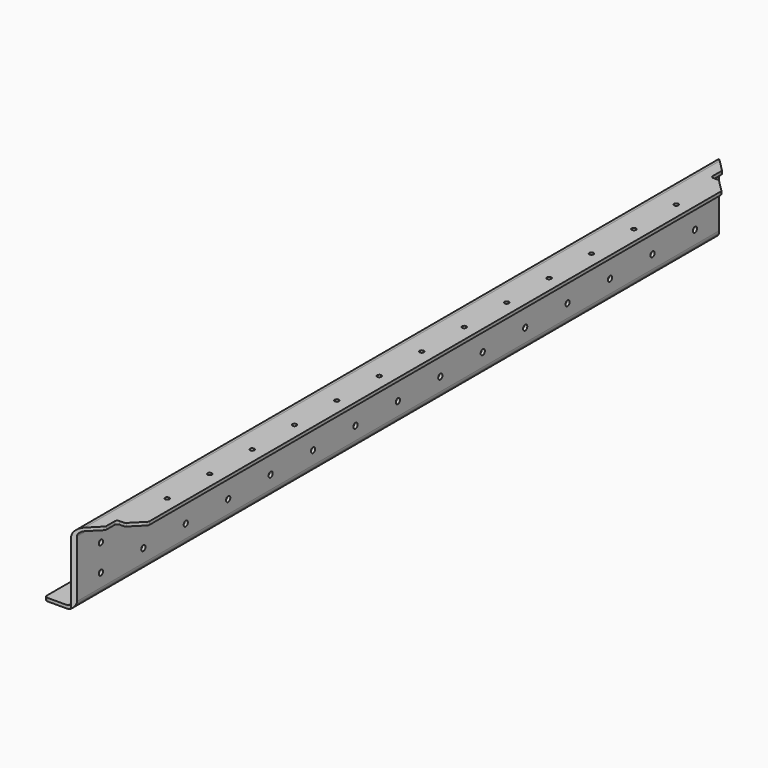
from build123d import *

# Parameters (mm, degrees)
F1_DEPTH    = 1525
F3_DEPTH    = 136.001
F4_R        = 8
F5_R        = 8
F6_R        = 14
F7_T1_DEPTH = 1583
F8_R        = 4.1
F9_DEPTH    = 136.001
F10_R       = 5
F11_DEPTH   = 76.001
F12_R       = 5
F13_DEPTH   = 6.001
F15_DEPTH   = 136.001
F16_R       = 5


# Not quite as in the source:
# - a fillet or chamfer that OpenCascade refuses, or shapes differently, is made with other operations: its cross-section is extruded or revolved along the edge and cut away or added
# - two fillets or chamfers of one size are made in one step


with BuildPart() as f1:
    # F0 (on Front) → F1 (new body)
    with BuildSketch(Plane.XZ):
        Polygon((0, 130), (0, 0), (-50, 0), (-50, -6), (6, -6), (6, 124), (76, 124), (76, 130), align=None)
    extrude(amount=F1_DEPTH)

    # F2 (on face) → F3 (cut, through all)
    with BuildSketch(Plane.XY.offset(130)):
        Polygon((76, -76), (76, 0), (0, 0), align=None)
        Polygon((76, -1525), (76, -1449), (0, -1525), align=None)
    extrude(amount=-F3_DEPTH, mode=Mode.SUBTRACT)

    # F4
    f4_edges = [f1.edges().sort_by_distance(p)[0] for p in [
        (6, -762.5, 124),
    ]]
    fillet(f4_edges, radius=F4_R)

    # F5
    f5_edges = [f1.edges().sort_by_distance(p)[0] for p in [
        (0, -762.5, 0),
    ]]
    fillet(f5_edges, radius=F5_R)

    # F6
    f6_edges = [f1.edges().sort_by_distance(p)[0] for p in [
        (0, -762.5, 130),
    ]]
    fillet(f6_edges, radius=F6_R)

    # F7: fillet of radius 14 on 1 edges, made by hand

    # F7_s2 → F7_t1 (cut)
    with BuildSketch(Plane.XZ.offset(-29)):
        with BuildLine():
            ThreePointArc((-8, -6), (1.8994949366, -1.8994949366), (6, 8))
            Line((6, 8), (6, -6))
            Line((6, -6), (-8, -6))
        make_face()
    extrude(amount=F7_T1_DEPTH, mode=Mode.SUBTRACT)

    # F8 (on face) → F9 (cut, through all)
    with BuildSketch(Plane.XY.offset(130)):
        with Locations((51, -1362.5)):
            Circle(F8_R)
        with Locations((51, -1262.5)):
            Circle(F8_R)
        with Locations((51, -1162.5)):
            Circle(F8_R)
        with Locations((51, -1062.5)):
            Circle(F8_R)
        with Locations((51, -962.5)):
            Circle(F8_R)
        with Locations((51, -862.5)):
            Circle(F8_R)
        with Locations((51, -762.5)):
            Circle(F8_R)
        with Locations((51, -662.5)):
            Circle(F8_R)
        with Locations((51, -562.5)):
            Circle(F8_R)
        with Locations((51, -462.5)):
            Circle(F8_R)
        with Locations((51, -362.5)):
            Circle(F8_R)
        with Locations((51, -262.5)):
            Circle(F8_R)
        with Locations((51, -162.5)):
            Circle(F8_R)
    extrude(amount=-F9_DEPTH, mode=Mode.SUBTRACT)

    # F10 (on face) → F11 (cut, through all)
    with BuildSketch(Plane(origin=(0, 0, 0), x_dir=(0, -1, 0), z_dir=(-1, 0, 0))):
        with Locations((1462.5, 33)):
            Circle(F10_R)
        with Locations((1362.5, 33)):
            Circle(F10_R)
        with Locations((1262.5, 33)):
            Circle(F10_R)
        with Locations((1162.5, 33)):
            Circle(F10_R)
        with Locations((1062.5, 33)):
            Circle(F10_R)
        with Locations((962.5, 33)):
            Circle(F10_R)
        with Locations((862.5, 33)):
            Circle(F10_R)
        with Locations((762.5, 33)):
            Circle(F10_R)
        with Locations((662.5, 33)):
            Circle(F10_R)
        with Locations((562.5, 33)):
            Circle(F10_R)
        with Locations((462.5, 33)):
            Circle(F10_R)
        with Locations((362.5, 33)):
            Circle(F10_R)
        with Locations((262.5, 33)):
            Circle(F10_R)
        with Locations((162.5, 33)):
            Circle(F10_R)
        with Locations((62.5, 33)):
            Circle(F10_R)
        with Locations((1462.5, 83)):
            Circle(F10_R)
        with Locations((1362.5, 83)):
            Circle(F10_R)
        with Locations((1262.5, 83)):
            Circle(F10_R)
        with Locations((1162.5, 83)):
            Circle(F10_R)
        with Locations((1062.5, 83)):
            Circle(F10_R)
        with Locations((962.5, 83)):
            Circle(F10_R)
        with Locations((862.5, 83)):
            Circle(F10_R)
        with Locations((462.5, 83)):
            Circle(F10_R)
        with Locations((562.5, 83)):
            Circle(F10_R)
        with Locations((662.5, 83)):
            Circle(F10_R)
        with Locations((762.5, 83)):
            Circle(F10_R)
        with Locations((162.5, 83)):
            Circle(F10_R)
        with Locations((262.5, 83)):
            Circle(F10_R)
        with Locations((62.5, 83)):
            Circle(F10_R)
        with Locations((362.5, 83)):
            Circle(F10_R)
    extrude(amount=-F11_DEPTH, mode=Mode.SUBTRACT)

    # F12 (on face) → F13 (cut, through all)
    with BuildSketch(Plane.XY):
        with Locations((-25, -1462.5)):
            Circle(F12_R)
        with Locations((-25, -1362.5)):
            Circle(F12_R)
        with Locations((-25, -1262.5)):
            Circle(F12_R)
        with Locations((-25, -1162.5)):
            Circle(F12_R)
        with Locations((-25, -1062.5)):
            Circle(F12_R)
        with Locations((-25, -962.5)):
            Circle(F12_R)
        with Locations((-25, -862.5)):
            Circle(F12_R)
        with Locations((-25, -762.5)):
            Circle(F12_R)
        with Locations((-25, -662.5)):
            Circle(F12_R)
        with Locations((-25, -562.5)):
            Circle(F12_R)
        with Locations((-25, -462.5)):
            Circle(F12_R)
        with Locations((-25, -362.5)):
            Circle(F12_R)
        with Locations((-25, -262.5)):
            Circle(F12_R)
        with Locations((-25, -162.5)):
            Circle(F12_R)
        with Locations((-25, -62.5)):
            Circle(F12_R)
    extrude(amount=-F13_DEPTH, mode=Mode.SUBTRACT)

    # F14 (on face) → F15 (cut, through all)
    with BuildSketch(Plane.XY.offset(130)):
        Polygon((76, -76), (36, -36), (36, -62.5), (51.186291501, -62.5), (76, -87.313708499), align=None)
        Polygon((36, -1462.5), (36, -1489), (76, -1449), (76, -1437.686291501), (51.186291501, -1462.5), align=None)
    extrude(amount=-F15_DEPTH, mode=Mode.SUBTRACT)

    # F16
    f16_edges = [f1.edges().sort_by_distance(p)[0] for p in [
        (36, -36, 127),
        (36, -62.5, 127),
        (36, -1489, 127),
        (36, -1462.5, 127),
        (51.186292, -62.5, 127),
        (76, -87.313708, 127),
        (51.186292, -1462.5, 127),
        (76, -1437.686292, 127),
        (-50, 0, -3),
        (-50, -1525, -3),
    ]]
    fillet(f16_edges, radius=F16_R)


solid = f1.part
